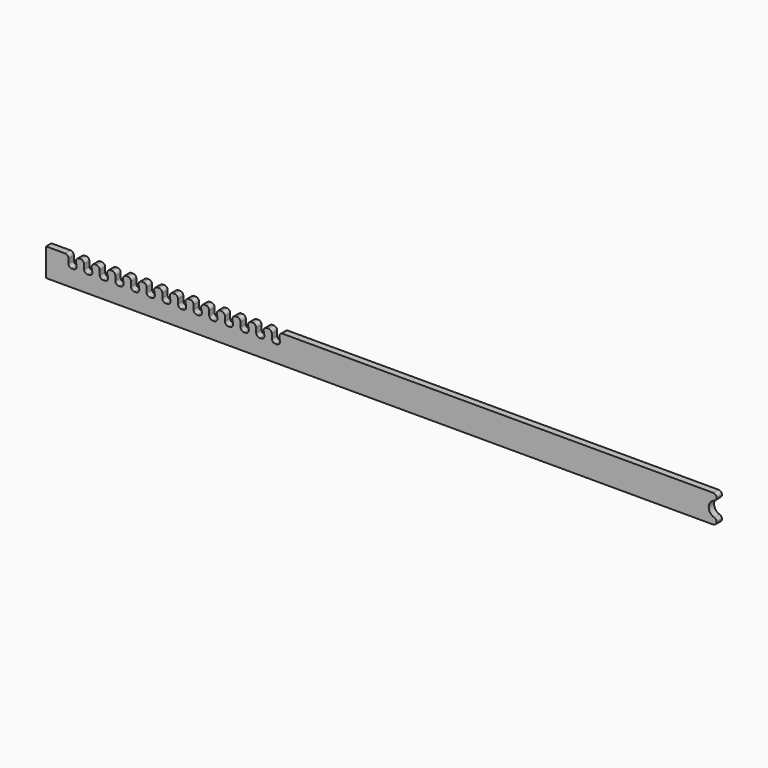
from build123d import *

# Parameters (mm, degrees)
F1_DEPTH    = 6
F2_T1_DEPTH = 6
F2_T3_DEPTH = 24.523457348
F2_T5_DEPTH = 21
F2_T7_DEPTH = 18.6969600709


# Not quite as in the source:
# - a fillet or chamfer that OpenCascade refuses, or shapes differently, is made with other operations: its cross-section is extruded or revolved along the edge and cut away or added


with BuildPart() as f1:
    # F0 (on Front) → F1 (new body)
    with BuildSketch(Plane.XZ):
        with BuildLine():
            Line((0, 25), (0, 0))
            Line((0, 0), (600, 0))
            Line((600, 0), (600, 5.5))
            ThreePointArc((600, 5.5), (593, 12.5), (600, 19.5))
            Line((600, 19.5), (600, 25))
            Line((600, 25), (208, 25))
            Line((208, 25), (210.1255656167, 15))
            Line((210.1255656167, 15), (208, 15))
            Line((208, 15), (202, 15))
            Line((202, 15), (202, 25))
            Line((202, 25), (194, 25))
            Line((194, 25), (196.1255656167, 15))
            Line((196.1255656167, 15), (194, 15))
            Line((194, 15), (188, 15))
            Line((188, 15), (188, 25))
            Line((188, 25), (180, 25))
            Line((180, 25), (182.1255656167, 15))
            Line((182.1255656167, 15), (180, 15))
            Line((180, 15), (174, 15))
            Line((174, 15), (174, 25))
            Line((174, 25), (166, 25))
            Line((166, 25), (168.1255656167, 15))
            Line((168.1255656167, 15), (166, 15))
            Line((166, 15), (160, 15))
            Line((160, 15), (160, 25))
            Line((160, 25), (152, 25))
            Line((152, 25), (154.1255656167, 15))
            Line((154.1255656167, 15), (152, 15))
            Line((152, 15), (146, 15))
            Line((146, 15), (146, 25))
            Line((146, 25), (138, 25))
            Line((138, 25), (140.1255656167, 15))
            Line((140.1255656167, 15), (138, 15))
            Line((138, 15), (132, 15))
            Line((132, 15), (132, 25))
            Line((132, 25), (124, 25))
            Line((124, 25), (126.1255656167, 15))
            Line((126.1255656167, 15), (124, 15))
            Line((124, 15), (118, 15))
            Line((118, 15), (118, 25))
            Line((118, 25), (110, 25))
            Line((110, 25), (112.1255656167, 15))
            Line((112.1255656167, 15), (110, 15))
            Line((110, 15), (104, 15))
            Line((104, 15), (104, 25))
            Line((104, 25), (96, 25))
            Line((96, 25), (98.1255656167, 15))
            Line((98.1255656167, 15), (96, 15))
            Line((96, 15), (90, 15))
            Line((90, 15), (90, 25))
            Line((90, 25), (82, 25))
            Line((82, 25), (84.1255656167, 15))
            Line((84.1255656167, 15), (82, 15))
            Line((82, 15), (76, 15))
            Line((76, 15), (76, 25))
            Line((76, 25), (68, 25))
            Line((68, 25), (70.1255656167, 15))
            Line((70.1255656167, 15), (68, 15))
            Line((68, 15), (62, 15))
            Line((62, 15), (62, 25))
            Line((62, 25), (54, 25))
            Line((54, 25), (56.1255656167, 15))
            Line((56.1255656167, 15), (54, 15))
            Line((54, 15), (48, 15))
            Line((48, 15), (48, 25))
            Line((48, 25), (40, 25))
            Line((40, 25), (42.1255656167, 15))
            Line((42.1255656167, 15), (40, 15))
            Line((40, 15), (34, 15))
            Line((34, 15), (34, 25))
            Line((34, 25), (26, 25))
            Line((26, 25), (28.1255656167, 15))
            Line((28.1255656167, 15), (26, 15))
            Line((26, 15), (20, 15))
            Line((20, 15), (20, 25))
            Line((20, 25), (0, 25))
        make_face()
    extrude(amount=F1_DEPTH)

    # F2: fillet of radius 3 on 60 edges, made by hand

    # F2_s2 → F2_t1 (join)
    with BuildSketch(Plane.XZ):
        with BuildLine():
            ThreePointArc((20, 18), (20.8786796564, 15.8786796564), (23, 15))
            Line((23, 15), (20, 15))
            Line((20, 15), (20, 18))
        make_face()
        with BuildLine():
            ThreePointArc((37, 15), (34.8786796564, 15.8786796564), (34, 18))
            Line((34, 18), (34, 15))
            Line((34, 15), (37, 15))
        make_face()
        with BuildLine():
            ThreePointArc((48, 18), (48.8786796564, 15.8786796564), (51, 15))
            Line((51, 15), (48, 15))
            Line((48, 15), (48, 18))
        make_face()
        with BuildLine():
            ThreePointArc((62, 18), (62.8786796564, 15.8786796564), (65, 15))
            Line((65, 15), (62, 15))
            Line((62, 15), (62, 18))
        make_face()
        with BuildLine():
            ThreePointArc((76, 18), (76.8786796564, 15.8786796564), (79, 15))
            Line((79, 15), (76, 15))
            Line((76, 15), (76, 18))
        make_face()
        with BuildLine():
            ThreePointArc((90, 18), (90.8786796564, 15.8786796564), (93, 15))
            Line((93, 15), (90, 15))
            Line((90, 15), (90, 18))
        make_face()
        with BuildLine():
            ThreePointArc((104, 18), (104.8786796564, 15.8786796564), (107, 15))
            Line((107, 15), (104, 15))
            Line((104, 15), (104, 18))
        make_face()
        with BuildLine():
            ThreePointArc((118, 18), (118.8786796564, 15.8786796564), (121, 15))
            Line((121, 15), (118, 15))
            Line((118, 15), (118, 18))
        make_face()
        with BuildLine():
            ThreePointArc((132, 18), (132.8786796564, 15.8786796564), (135, 15))
            Line((135, 15), (132, 15))
            Line((132, 15), (132, 18))
        make_face()
        with BuildLine():
            ThreePointArc((146, 18), (146.8786796564, 15.8786796564), (149, 15))
            Line((149, 15), (146, 15))
            Line((146, 15), (146, 18))
        make_face()
        with BuildLine():
            ThreePointArc((160, 18), (160.8786796564, 15.8786796564), (163, 15))
            Line((163, 15), (160, 15))
            Line((160, 15), (160, 18))
        make_face()
        with BuildLine():
            ThreePointArc((174, 18), (174.8786796564, 15.8786796564), (177, 15))
            Line((177, 15), (174, 15))
            Line((174, 15), (174, 18))
        make_face()
        with BuildLine():
            ThreePointArc((188, 18), (188.8786796564, 15.8786796564), (191, 15))
            Line((191, 15), (188, 15))
            Line((188, 15), (188, 18))
        make_face()
        with BuildLine():
            ThreePointArc((202, 18), (202.8786796564, 15.8786796564), (205, 15))
            Line((205, 15), (202, 15))
            Line((202, 15), (202, 18))
        make_face()
        with BuildLine():
            ThreePointArc((24.4208741471, 15), (26.7523120315, 16.1120388269), (27.3553169493, 18.6237350725))
            Line((27.3553169493, 18.6237350725), (28.1255656167, 15))
            Line((28.1255656167, 15), (24.4208741471, 15))
        make_face()
        with BuildLine():
            ThreePointArc((38.4208741471, 15), (40.7523120315, 16.1120388269), (41.3553169493, 18.6237350725))
            Line((41.3553169493, 18.6237350725), (42.1255656167, 15))
            Line((42.1255656167, 15), (38.4208741471, 15))
        make_face()
        with BuildLine():
            ThreePointArc((52.4208741471, 15), (54.7523120315, 16.1120388269), (55.3553169493, 18.6237350725))
            Line((55.3553169493, 18.6237350725), (56.1255656167, 15))
            Line((56.1255656167, 15), (52.4208741471, 15))
        make_face()
        with BuildLine():
            ThreePointArc((66.4208741471, 15), (68.7523120315, 16.1120388269), (69.3553169493, 18.6237350725))
            Line((69.3553169493, 18.6237350725), (70.1255656167, 15))
            Line((70.1255656167, 15), (66.4208741471, 15))
        make_face()
        with BuildLine():
            ThreePointArc((80.4208741471, 15), (82.7523120315, 16.1120388269), (83.3553169493, 18.6237350725))
            Line((83.3553169493, 18.6237350725), (84.1255656167, 15))
            Line((84.1255656167, 15), (80.4208741471, 15))
        make_face()
        with BuildLine():
            ThreePointArc((94.4208741471, 15), (96.7523120315, 16.1120388269), (97.3553169493, 18.6237350725))
            Line((97.3553169493, 18.6237350725), (98.1255656167, 15))
            Line((98.1255656167, 15), (94.4208741471, 15))
        make_face()
        with BuildLine():
            ThreePointArc((108.4208741471, 15), (110.7523120315, 16.1120388269), (111.3553169493, 18.6237350725))
            Line((111.3553169493, 18.6237350725), (112.1255656167, 15))
            Line((112.1255656167, 15), (108.4208741471, 15))
        make_face()
        with BuildLine():
            ThreePointArc((122.4208741471, 15), (124.7523120315, 16.1120388269), (125.3553169493, 18.6237350725))
            Line((125.3553169493, 18.6237350725), (126.1255656167, 15))
            Line((126.1255656167, 15), (122.4208741471, 15))
        make_face()
        with BuildLine():
            ThreePointArc((136.4208741471, 15), (138.7523120315, 16.1120388269), (139.3553169493, 18.6237350725))
            Line((139.3553169493, 18.6237350725), (140.1255656167, 15))
            Line((140.1255656167, 15), (136.4208741471, 15))
        make_face()
        with BuildLine():
            ThreePointArc((150.4208741471, 15), (152.7523120315, 16.1120388269), (153.3553169493, 18.6237350725))
            Line((153.3553169493, 18.6237350725), (154.1255656167, 15))
            Line((154.1255656167, 15), (150.4208741471, 15))
        make_face()
        with BuildLine():
            ThreePointArc((164.4208741471, 15), (166.7523120315, 16.1120388269), (167.3553169493, 18.6237350725))
            Line((167.3553169493, 18.6237350725), (168.1255656167, 15))
            Line((168.1255656167, 15), (164.4208741471, 15))
        make_face()
        with BuildLine():
            ThreePointArc((178.4208741471, 15), (180.7523120315, 16.1120388269), (181.3553169493, 18.6237350725))
            Line((181.3553169493, 18.6237350725), (182.1255656167, 15))
            Line((182.1255656167, 15), (178.4208741471, 15))
        make_face()
        with BuildLine():
            ThreePointArc((192.4208741471, 15), (194.7523120315, 16.1120388269), (195.3553169493, 18.6237350725))
            Line((195.3553169493, 18.6237350725), (196.1255656167, 15))
            Line((196.1255656167, 15), (192.4208741471, 15))
        make_face()
        with BuildLine():
            ThreePointArc((206.4208741471, 15), (208.7523120315, 16.1120388269), (209.3553169493, 18.6237350725))
            Line((209.3553169493, 18.6237350725), (210.1255656167, 15))
            Line((210.1255656167, 15), (206.4208741471, 15))
        make_face()
    extrude(amount=F2_T1_DEPTH)

    # F2_s4 → F2_t3 (cut)
    with BuildSketch(Plane.XZ.offset(-9.261728674)):
        with BuildLine():
            ThreePointArc((29.7046914696, 25), (27.3732535852, 23.8879611731), (26.7702486674, 21.3762649275))
            Line((26.7702486674, 21.3762649275), (26, 25))
            Line((26, 25), (29.7046914696, 25))
        make_face()
        with BuildLine():
            ThreePointArc((43.7046914696, 25), (41.3732535852, 23.8879611731), (40.7702486674, 21.3762649275))
            Line((40.7702486674, 21.3762649275), (40, 25))
            Line((40, 25), (43.7046914696, 25))
        make_face()
        with BuildLine():
            ThreePointArc((57.7046914696, 25), (55.3732535852, 23.8879611731), (54.7702486674, 21.3762649275))
            Line((54.7702486674, 21.3762649275), (54, 25))
            Line((54, 25), (57.7046914696, 25))
        make_face()
        with BuildLine():
            ThreePointArc((71.7046914696, 25), (69.3732535852, 23.8879611731), (68.7702486674, 21.3762649275))
            Line((68.7702486674, 21.3762649275), (68, 25))
            Line((68, 25), (71.7046914696, 25))
        make_face()
        with BuildLine():
            ThreePointArc((85.7046914696, 25), (83.3732535852, 23.8879611731), (82.7702486674, 21.3762649275))
            Line((82.7702486674, 21.3762649275), (82, 25))
            Line((82, 25), (85.7046914696, 25))
        make_face()
        with BuildLine():
            ThreePointArc((99.7046914696, 25), (97.3732535852, 23.8879611731), (96.7702486674, 21.3762649275))
            Line((96.7702486674, 21.3762649275), (96, 25))
            Line((96, 25), (99.7046914696, 25))
        make_face()
        with BuildLine():
            ThreePointArc((113.7046914696, 25), (111.3732535852, 23.8879611731), (110.7702486674, 21.3762649275))
            Line((110.7702486674, 21.3762649275), (110, 25))
            Line((110, 25), (113.7046914696, 25))
        make_face()
        with BuildLine():
            ThreePointArc((127.7046914696, 25), (125.3732535852, 23.8879611731), (124.7702486674, 21.3762649275))
            Line((124.7702486674, 21.3762649275), (124, 25))
            Line((124, 25), (127.7046914696, 25))
        make_face()
        with BuildLine():
            ThreePointArc((141.7046914696, 25), (139.3732535852, 23.8879611731), (138.7702486674, 21.3762649275))
            Line((138.7702486674, 21.3762649275), (138, 25))
            Line((138, 25), (141.7046914696, 25))
        make_face()
        with BuildLine():
            ThreePointArc((155.7046914696, 25), (153.3732535852, 23.8879611731), (152.7702486674, 21.3762649275))
            Line((152.7702486674, 21.3762649275), (152, 25))
            Line((152, 25), (155.7046914696, 25))
        make_face()
        with BuildLine():
            ThreePointArc((169.7046914696, 25), (167.3732535852, 23.8879611731), (166.7702486674, 21.3762649275))
            Line((166.7702486674, 21.3762649275), (166, 25))
            Line((166, 25), (169.7046914696, 25))
        make_face()
        with BuildLine():
            ThreePointArc((183.7046914696, 25), (181.3732535852, 23.8879611731), (180.7702486674, 21.3762649275))
            Line((180.7702486674, 21.3762649275), (180, 25))
            Line((180, 25), (183.7046914696, 25))
        make_face()
        with BuildLine():
            ThreePointArc((197.7046914696, 25), (195.3732535852, 23.8879611731), (194.7702486674, 21.3762649275))
            Line((194.7702486674, 21.3762649275), (194, 25))
            Line((194, 25), (197.7046914696, 25))
        make_face()
        with BuildLine():
            ThreePointArc((211.7046914696, 25), (209.3732535852, 23.8879611731), (208.7702486674, 21.3762649275))
            Line((208.7702486674, 21.3762649275), (208, 25))
            Line((208, 25), (211.7046914696, 25))
        make_face()
    extrude(amount=F2_T3_DEPTH, mode=Mode.SUBTRACT)

    # F2_s6 → F2_t5 (cut)
    with BuildSketch(Plane.XZ.offset(-7.5)):
        with BuildLine():
            ThreePointArc((20, 22), (19.1213203436, 24.1213203436), (17, 25))
            Line((17, 25), (20, 25))
            Line((20, 25), (20, 22))
        make_face()
        with BuildLine():
            ThreePointArc((34, 22), (33.1213203436, 24.1213203436), (31, 25))
            Line((31, 25), (34, 25))
            Line((34, 25), (34, 22))
        make_face()
        with BuildLine():
            ThreePointArc((48, 22), (47.1213203436, 24.1213203436), (45, 25))
            Line((45, 25), (48, 25))
            Line((48, 25), (48, 22))
        make_face()
        with BuildLine():
            ThreePointArc((62, 22), (61.1213203436, 24.1213203436), (59, 25))
            Line((59, 25), (62, 25))
            Line((62, 25), (62, 22))
        make_face()
        with BuildLine():
            ThreePointArc((76, 22), (75.1213203436, 24.1213203436), (73, 25))
            Line((73, 25), (76, 25))
            Line((76, 25), (76, 22))
        make_face()
        with BuildLine():
            ThreePointArc((90, 22), (89.1213203436, 24.1213203436), (87, 25))
            Line((87, 25), (90, 25))
            Line((90, 25), (90, 22))
        make_face()
        with BuildLine():
            ThreePointArc((104, 22), (103.1213203436, 24.1213203436), (101, 25))
            Line((101, 25), (104, 25))
            Line((104, 25), (104, 22))
        make_face()
        with BuildLine():
            ThreePointArc((118, 22), (117.1213203436, 24.1213203436), (115, 25))
            Line((115, 25), (118, 25))
            Line((118, 25), (118, 22))
        make_face()
        with BuildLine():
            ThreePointArc((132, 22), (131.1213203436, 24.1213203436), (129, 25))
            Line((129, 25), (132, 25))
            Line((132, 25), (132, 22))
        make_face()
        with BuildLine():
            ThreePointArc((146, 22), (145.1213203436, 24.1213203436), (143, 25))
            Line((143, 25), (146, 25))
            Line((146, 25), (146, 22))
        make_face()
        with BuildLine():
            ThreePointArc((160, 22), (159.1213203436, 24.1213203436), (157, 25))
            Line((157, 25), (160, 25))
            Line((160, 25), (160, 22))
        make_face()
        with BuildLine():
            ThreePointArc((174, 22), (173.1213203436, 24.1213203436), (171, 25))
            Line((171, 25), (174, 25))
            Line((174, 25), (174, 22))
        make_face()
        with BuildLine():
            ThreePointArc((188, 22), (187.1213203436, 24.1213203436), (185, 25))
            Line((185, 25), (188, 25))
            Line((188, 25), (188, 22))
        make_face()
        with BuildLine():
            ThreePointArc((202, 22), (201.1213203436, 24.1213203436), (199, 25))
            Line((199, 25), (202, 25))
            Line((202, 25), (202, 22))
        make_face()
        with BuildLine():
            ThreePointArc((600, 22), (599.1213203436, 24.1213203436), (597, 25))
            Line((597, 25), (600, 25))
            Line((600, 25), (600, 22))
        make_face()
        with BuildLine():
            ThreePointArc((597, 0), (599.1213203436, 0.8786796564), (600, 3))
            Line((600, 3), (600, 0))
            Line((600, 0), (597, 0))
        make_face()
    extrude(amount=F2_T5_DEPTH, mode=Mode.SUBTRACT)

    # F2_s8 → F2_t7 (cut)
    with BuildSketch(Plane.XZ.offset(-6.3484800354)):
        with BuildLine():
            ThreePointArc((597.9, 19.1775744099), (599.4186773245, 20.2645680792), (600, 22.0393920142))
            Line((600, 22.0393920142), (600, 19.5))
            ThreePointArc((600, 19.5), (598.937696105, 19.4189240807), (597.9, 19.1775744099))
        make_face()
        with BuildLine():
            ThreePointArc((600, 2.9606079858), (599.4186773245, 4.7354319208), (597.9, 5.8224255901))
            ThreePointArc((597.9, 5.8224255901), (598.937696105, 5.5810759193), (600, 5.5))
            Line((600, 5.5), (600, 2.9606079858))
        make_face()
    extrude(amount=F2_T7_DEPTH, mode=Mode.SUBTRACT)


solid = f1.part
